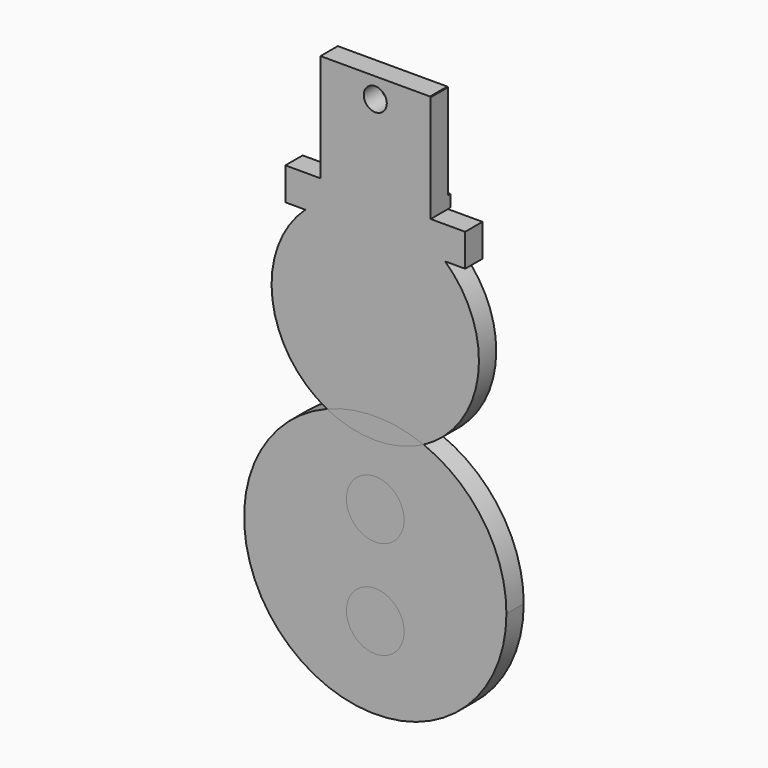
from build123d import *

# Parameters (mm, degrees)
F0_R          = 2.032
F0_R_2        = 3.81
F1_DEPTH      = 3.81
F0_R_3        = 5.08
F2_DEPTH      = 3.81
F3_DEPTH      = 2.54
F5_DEPTH      = 2.54
F6_DEPTH      = 2.54
F4_W          = 18.8897419721
F4_H          = 18.9798697829
F7_DEPTH      = 3.81
F9_DEPTH      = 0.508
F10_TEXT_SIZE = 4.8286410876
F11_DEPTH     = 0.635
F12_DEPTH     = 25.4


# Not quite as in the source:
# - a feature names something its author has since deleted; it is built from what else it names
# - Text() gives the source's letters only with a copy of the font that has no kerning and outlines rounded to 1/6400 em; it was checked with that copy


with BuildPart() as f1:
    # F0 (on Front) → F1 (new body)
    with BuildSketch(Plane.XZ):
        Polygon((-12.3248384371, 13.5021889186), (12.3248384371, 13.5021889186), (15.850013122, 13.5021889186), (15.850013122, 19.2414295611), (9.652, 19.2414295611), (9.652, 38.221299344), (-9.652, 38.221299344), (-9.652, 19.2425889186), (-15.850013122, 19.2425889186), (-15.850013122, 13.5021889186), align=None)
        with Locations((0, 34.6593298018)):
            Circle(F0_R, mode=Mode.SUBTRACT)
        with BuildLine():
            ThreePointArc((-8.5226943528, -16.1732627835), (0, -14.5454885481), (8.5226943528, -16.1732627835))
            ThreePointArc((8.5226943528, -16.1732627835), (18.1332019866, -2.3233023495), (12.3248384371, 13.5021889186))
            Line((12.3248384371, 13.5021889186), (-12.3248384371, 13.5021889186))
            ThreePointArc((-12.3248384371, 13.5021889186), (-18.1332019866, -2.3233023495), (-8.5226943528, -16.1732627835))
        make_face()
        with BuildLine():
            ThreePointArc((9.9695539102, -3.4508774988), (-0.3135427634, -10.0222190581), (-10.1967426017, -2.8635202907))
            Line((-10.1967426017, -2.8635202907), (-8.4882955998, -2.6387616526))
            ThreePointArc((-8.4882955998, -2.6387616526), (-0.3002245707, -8.7223650624), (8.2774581388, -3.2016679179))
            Line((8.2774581388, -3.2016679179), (9.9695539102, -3.4508774988))
        make_face(mode=Mode.SUBTRACT)
        with Locations((-8.2717526287, 6.7263835861)):
            Circle(F0_R_2, mode=Mode.SUBTRACT)
        with Locations((8.0187368014, 7.0260933531)):
            Circle(F0_R_2, mode=Mode.SUBTRACT)
    extrude(amount=-F1_DEPTH)

    # F0 (on Front) → F3 (join)
    with BuildSketch(Plane.XZ):
        with Locations((-8.2717526287, 6.7263835861)):
            Circle(F0_R_2)
        with Locations((8.0187368014, 7.0260933531)):
            Circle(F0_R_2)
    extrude(amount=-F3_DEPTH)

    # F0 (on Front) → F5 (join)
    with BuildSketch(Plane.XZ):
        with BuildLine():
            Line((-8.4882955998, -2.6387616526), (-10.1967426017, -2.8635202907))
            ThreePointArc((-10.1967426017, -2.8635202907), (-0.3135427634, -10.0222190581), (9.9695539102, -3.4508774988))
            Line((9.9695539102, -3.4508774988), (8.2774581388, -3.2016679179))
            ThreePointArc((8.2774581388, -3.2016679179), (-0.3002245707, -8.7223650624), (-8.4882955998, -2.6387616526))
        make_face()
    extrude(amount=-F5_DEPTH)

    # F4 (on Front) → F7 (join)
    with BuildSketch(Plane.XZ):
        with Locations((0.325685367, 28.6471430895)):
            Rectangle(F4_W, F4_H)
    extrude(amount=-F7_DEPTH)

    # F8 (on face) → F9 (join)
    with BuildSketch(Plane(origin=(0, 3.81, 0), x_dir=(-1, 0, 0), z_dir=(0, 1, 0))):
        Polygon((-9.770556353, 21.3839970529), (-9.770556353, 19.2414295611), (9.652, 19.2414295611), (9.652, 19.2425889186), (9.652, 21.3839970529), align=None)
    extrude(amount=F9_DEPTH)

    # F10 (on face) → F11 (cut)
    with BuildSketch(Plane(origin=(0, 3.81, 0), x_dir=(-1, 0, 0), z_dir=(0, 1, 0))):
        with Locations((-11.5569159389, 14.673339203)):
            Text('SSEC 2016', F10_TEXT_SIZE, font='Open Sans', text_align=(TextAlign.LEFT, TextAlign.BOTTOM))
    extrude(amount=-F11_DEPTH, mode=Mode.SUBTRACT)

    # F0 (on Front) → F12 (cut)
    with BuildSketch(Plane.XZ):
        with Locations((0, 34.6593298018)):
            Circle(F0_R)
    extrude(amount=-F12_DEPTH, mode=Mode.SUBTRACT)


with BuildPart() as f1b:
    # F0 (on Front) → F1, piece 2 (new body)
    with BuildSketch(Plane.XZ):
        with BuildLine():
            ThreePointArc((-8.5226943528, -16.1732627835), (-12.9941266286, -56.8004360069), (23.1254329861, -37.6709215343))
            ThreePointArc((23.1254329861, -37.6709215343), (19.1295144726, -24.6767949057), (8.5226943528, -16.1732627835))
            ThreePointArc((8.5226943528, -16.1732627835), (0, -18.2814317846), (-8.5226943528, -16.1732627835))
        make_face()
        with Locations((0, -46.3437545204)):
            Circle(F0_R_3, mode=Mode.SUBTRACT)
        with Locations((0, -28.9859827608)):
            Circle(F0_R_3, mode=Mode.SUBTRACT)
    extrude(amount=-F1_DEPTH)


with BuildPart() as f2:
    # F0 (on Front) → F2 (new body)
    with BuildSketch(Plane.XZ):
        with BuildLine():
            ThreePointArc((-8.5226943528, -16.1732627835), (0, -18.2814317846), (8.5226943528, -16.1732627835))
            ThreePointArc((8.5226943528, -16.1732627835), (0, -14.5454885481), (-8.5226943528, -16.1732627835))
        make_face()
    extrude(amount=-F2_DEPTH)


with BuildPart() as f6:
    # F0 (on Front) → F6 (new body)
    with BuildSketch(Plane.XZ):
        with Locations((0, -46.3437545204)):
            Circle(F0_R_3)
    extrude(amount=-F6_DEPTH)


with BuildPart() as f6b:
    # F0 (on Front) → F6, piece 2 (new body)
    with BuildSketch(Plane.XZ):
        with Locations((0, -28.9859827608)):
            Circle(F0_R_3)
    extrude(amount=-F6_DEPTH)


solid = Compound([f1.part, f1b.part, f2.part, f6.part, f6b.part])
